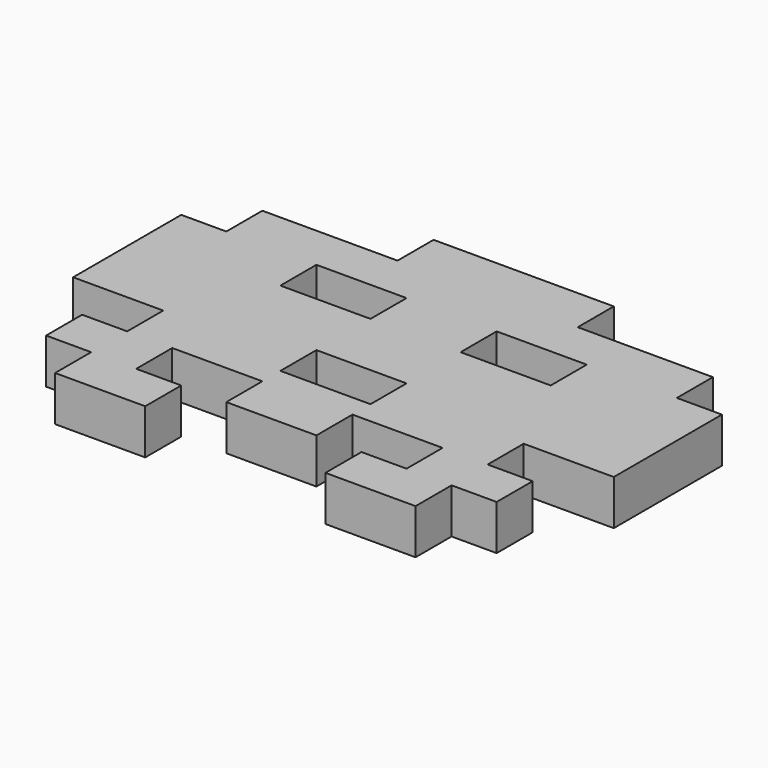
from build123d import *

# Parameters (mm, degrees)
F0_R     = 6
F1_DEPTH = 10
F3_DEPTH = 3


with BuildPart() as f1:
    # F0 (on Top) → F1 (new body)
    with BuildSketch(Plane.XY):
        Polygon((10, 0), (0, 0), (-10, 0), (-20, 0), (-20, -10), (-30, -10), (-40, -10), (-50, -10), (-50, -20), (-60, -20), (-60, -30), (-60, -40), (-60, -50), (-50, -50), (-40, -50), (-40, -60), (-50, -60), (-50, -70), (-40, -70), (-40, -80), (-30, -80), (-20, -80), (-20, -70), (-30, -70), (-30, -60), (-20, -60), (-10, -60), (-10, -70), (0, -70), (10, -70), (10, -60), (20, -60), (30, -60), (30, -70), (20, -70), (20, -80), (30, -80), (40, -80), (40, -70), (50, -70), (50, -60), (40, -60), (40, -50), (50, -50), (60, -50), (60, -40), (60, -30), (60, -20), (50, -20), (50, -10), (40, -10), (30, -10), (20, -10), (20, 0), align=None)
        Polygon((-10, -45), (0, -45), (10, -45), (10, -55), (0, -55), (-10, -55), align=None, mode=Mode.SUBTRACT)
        Polygon((-30, -30), (-30, -20), (-20, -20), (-10, -20), (-10, -30), (-20, -30), align=None, mode=Mode.SUBTRACT)
        Polygon((10, -20), (20, -20), (30, -20), (30, -30), (20, -30), (10, -30), align=None, mode=Mode.SUBTRACT)
        with Locations((0, -12)):
            Circle(F0_R, mode=Mode.SUBTRACT)
        with Locations((0, -12)):
            Circle(F0_R)
    extrude(amount=F1_DEPTH)

    # F2 (on Right) → F3 (cut, symmetric)
    with BuildSketch(Plane.YZ):
        Polygon((-16, 5), (-16, 0), (-10, 0), (-7.1132486541, 5), align=None)
    extrude(amount=F3_DEPTH, both=True, mode=Mode.SUBTRACT)


solid = f1.part
